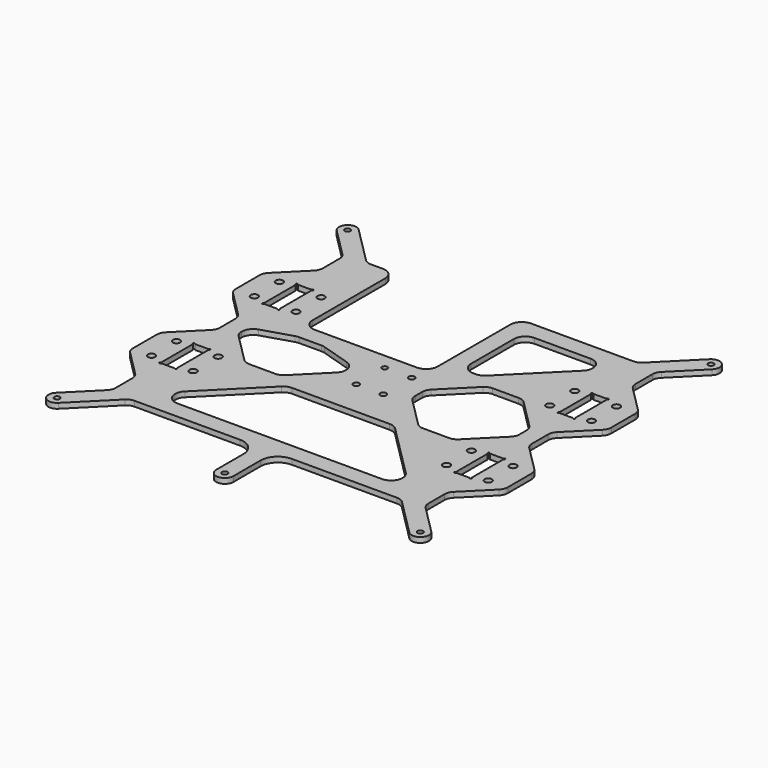
from build123d import *

# Parameters (mm, degrees)
F0_R     = 1.6
F0_R_2   = 2.1
F0_R_3   = 1.75
F1_DEPTH = 3


# Not quite as in the source:
# - ends of sketch curves that miss each other by under 0.0002 mm in the source are joined


with BuildPart() as f1:
    # F0 (on Top) → F1 (new body)
    with BuildSketch(Plane.XY):
        with BuildLine():
            Line((-91.7573578066, 64.2426430438), (-106.2426418066, 49.7573620438))
            ThreePointArc((-106.2426418066, 49.7573620438), (-107.5432800387, 47.8108195211), (-108.0000028014, 45.5147184321))
            Line((-108.0000028014, 45.5147184321), (-108.0000028014, 28.4852814321))
            ThreePointArc((-108.0000028014, 28.4852814321), (-107.5432780557, 26.1891807819), (-106.2426416956, 24.2426405379))
            Line((-106.2426416956, 24.2426405379), (-91.7573578066, 9.7573586489))
            ThreePointArc((-91.7573578066, 9.7573586489), (-90.4567263652, 7.8108163857), (-90.000004, 5.5147176489))
            Line((-90.000004, 5.5147176489), (-90.000004, -5.5147181357))
            ThreePointArc((-90.000004, -5.5147181357), (-90.4567266866, -7.810818842), (-91.7573628987, -9.7573592371))
            Line((-91.7573628987, -9.7573592371), (-106.2426418014, -24.2426401357))
            ThreePointArc((-106.2426418014, -24.2426401357), (-107.5432798474, -26.1891795848), (-108.0000028014, -28.4852801357))
            Line((-108.0000028014, -28.4852801357), (-108.0000028014, -45.5147181357))
            ThreePointArc((-108.0000028014, -45.5147181357), (-107.5432780557, -47.810818786), (-106.2426416956, -49.75735903))
            Line((-106.2426416956, -49.75735903), (-91.7573578014, -64.2426391357))
            ThreePointArc((-91.7573578014, -64.2426391357), (-90.4567259825, -66.1891833228), (-90.000004, -68.4852831357))
            Line((-90.000004, -68.4852831357), (-90.000004, -80.514722))
            ThreePointArc((-90.000004, -80.514722), (-90.4567219139, -82.8108200561), (-91.7573566058, -84.7573583942))
            Line((-91.7573566058, -84.7573583942), (-108.000003, -101.000004))
            ThreePointArc((-108.000003, -101.000004), (-107.9999999189, -107.9999994189), (-101.0000038311, -108.0000031689))
            Line((-101.0000038311, -108.0000031689), (-79.757363, -86.757362))
            ThreePointArc((-79.757363, -86.757362), (-77.8108216333, -85.4567247319), (-75.51472, -85.000001))
            Line((-75.51472, -85.000001), (-14.949748, -85.000001))
            ThreePointArc((-14.949748, -85.000001), (-7.8786801881, -87.9289331881), (-4.949748, -95.000001))
            Line((-4.949748, -95.000001), (-4.949747, -114.500004))
            ThreePointArc((-4.949747, -114.500004), (0, -119.449747), (4.949747, -114.500004))
            Line((4.949747, -114.500004), (4.949746, -95.000001))
            ThreePointArc((4.949746, -95.000001), (7.8786781881, -87.9289331881), (14.949746, -85.000001))
            Line((14.949746, -85.000001), (75.514718, -85.000001))
            ThreePointArc((75.514718, -85.000001), (77.8108209367, -85.4567226928), (79.7573623942, -86.7573616058))
            Line((79.7573623942, -86.7573616058), (101.000003, -108.000003))
            ThreePointArc((101.000003, -108.000003), (107.9999999189, -107.9999994189), (108.0000021689, -101.0000028311))
            Line((108.0000021689, -101.0000028311), (91.757279, -84.757281))
            ThreePointArc((91.757279, -84.757281), (90.4566428049, -82.8107405942), (89.99992, -80.51464))
            Line((89.99992, -80.51464), (89.99992, -68.9356846639))
            ThreePointArc((89.99992, -68.9356846639), (90.4566436949, -66.6395847167), (91.7572811413, -64.6930458052))
            Line((91.7572811413, -64.6930458052), (106.2425711968, -50.2077726639))
            ThreePointArc((106.2425711968, -50.2077726639), (107.5432095472, -48.2612339103), (107.9999341968, -45.9651336639))
            Line((107.9999341968, -45.9651336639), (107.9999501968, -28.9356956639))
            ThreePointArc((107.9999501968, -28.9356956639), (107.5432290112, -26.6395943825), (106.2425940052, -24.6930528554))
            Line((106.2425940052, -24.6930528554), (91.7573201968, -10.2077616639))
            ThreePointArc((91.7573201968, -10.2077616639), (90.4566900386, -8.261219774), (89.9999692559, -5.9651186639))
            Line((89.9999692559, -5.9651186639), (89.999978386, 5.514733204))
            ThreePointArc((89.999978386, 5.514733204), (90.4567025196, 7.8108314385), (91.7573390273, 9.7573687908))
            Line((91.7573390273, 9.7573687908), (106.2426308014, 24.2426424321))
            ThreePointArc((106.2426308014, 24.2426424321), (107.5432689605, 26.1891807238), (107.9999938014, 28.4852804321))
            Line((107.9999938014, 28.4852804321), (108.0000098014, 45.5147194321))
            ThreePointArc((108.0000098014, 45.5147194321), (107.5432888072, 47.8108202515), (106.2426536099, 49.7573622406))
            Line((106.2426536099, 49.7573622406), (91.7573798014, 64.2426534321))
            ThreePointArc((91.7573798014, 64.2426534321), (90.4567425354, 66.1891959193), (90.000022, 68.4852984321))
            Line((90.000022, 68.4852984321), (90.000022, 80.514742))
            ThreePointArc((90.000022, 80.514742), (90.4567448049, 82.8108425942), (91.7573813129, 84.7573826871))
            Line((91.7573813129, 84.7573826871), (108.000002, 101.000003))
            ThreePointArc((108.000002, 101.000003), (107.9999996689, 107.9999996689), (101.0000033311, 108.0000026689))
            Line((101.0000033311, 108.0000026689), (79.757362, 86.757362))
            ThreePointArc((79.757362, 86.757362), (77.8108201714, 85.4567245406), (75.514718, 85.000001))
            Line((75.514718, 85.000001), (16.5999989614, 85.000001))
            ThreePointArc((16.5999989614, 85.000001), (11.933094179, 83.0669057293), (9.9999989614, 78.400000925))
            Line((9.9999989614, 78.400000925), (9.9999993466, 26.100000075))
            ThreePointArc((9.9999993466, 26.100000075), (8.0669041289, 21.4330952707), (3.3999993466, 19.5))
            Line((3.3999993466, 19.5), (-55.3999990225, 19.5))
            ThreePointArc((-55.3999990225, 19.5), (-60.0669037518, 21.4330952177), (-61.9999990225, 26.099999925))
            Line((-61.9999990225, 26.099999925), (-61.9999996168, 78.3999997378))
            ThreePointArc((-61.9999996168, 78.3999997378), (-63.9330951112, 83.0669046688), (-68.6000002494, 84.9999996628))
            Line((-68.6000002494, 84.9999996628), (-75.5147185782, 84.999999))
            ThreePointArc((-75.5147185782, 84.999999), (-77.8108213035, 85.4567230195), (-79.7573624724, 86.7573621058))
            Line((-79.7573624724, 86.7573621058), (-101.000004, 108.000003))
            ThreePointArc((-101.000004, 108.000003), (-107.9999996689, 107.9999996689), (-108.0000031689, 101.0000038311))
            Line((-108.0000031689, 101.0000038311), (-91.757358, 84.757358))
            ThreePointArc((-91.757358, 84.757358), (-90.4567266686, 82.8108174694), (-90.000004, 80.514721))
            Line((-90.000004, 80.514721), (-90.000004, 68.4852860438))
            ThreePointArc((-90.000004, 68.4852860438), (-90.4567264392, 66.1891839348), (-91.7573578066, 64.2426430438))
        make_face()
        with Locations((-104.5, -104.5)):
            Circle(F0_R, mode=Mode.SUBTRACT)
        with Locations((-97, -45.9999990463)):
            Circle(F0_R_2, mode=Mode.SUBTRACT)
        with BuildLine():
            Line((-81.3660647171, -49.0500016357), (-88.6340257171, -49.0499986357))
            ThreePointArc((-88.6340257171, -49.0499986357), (-88.8840255651, -49.1169858461), (-89.0670382435, -49.2999983318))
            ThreePointArc((-89.0670382435, -49.2999983318), (-89.8536046247, -49.4035525093), (-89.750052771, -48.6169865423))
            ThreePointArc((-89.750052771, -48.6169865423), (-89.5670414944, -48.4339747338), (-89.5000547171, -48.1839756357))
            Line((-89.5000547171, -48.1839756357), (-89.5000547171, -25.8160226357))
            ThreePointArc((-89.5000547171, -25.8160226357), (-89.5670414944, -25.5660235377), (-89.7500529131, -25.3830109753))
            ThreePointArc((-89.7500529131, -25.3830109753), (-89.8536046247, -24.5964447622), (-89.0670389406, -24.6999987648))
            ThreePointArc((-89.0670389406, -24.6999987648), (-88.8840255651, -24.8830114254), (-88.6340257171, -24.9499986357))
            Line((-88.6340257171, -24.9499986357), (-81.3660647171, -24.9499956357))
            ThreePointArc((-81.3660647171, -24.9499956357), (-81.116065244, -24.8830086419), (-80.9330526237, -24.6999966897))
            ThreePointArc((-80.9330526237, -24.6999966897), (-80.1464875373, -24.5964460343), (-80.2500418461, -25.3830114122))
            ThreePointArc((-80.2500418461, -25.3830114122), (-80.4330543817, -25.5660245712), (-80.5000417171, -25.8160246357))
            Line((-80.5000417171, -25.8160246357), (-80.5000417171, -48.1839736357))
            ThreePointArc((-80.5000417171, -48.1839736357), (-80.4330543817, -48.4339737003), (-80.250041588, -48.6169864122))
            ThreePointArc((-80.250041588, -48.6169864122), (-80.1464878435, -49.4035515434), (-80.9330538105, -49.2999996897))
            ThreePointArc((-80.9330538105, -49.2999996897), (-81.116065619, -49.1169884131), (-81.3660647171, -49.0500016357))
        make_face(mode=Mode.SUBTRACT)
        with Locations((-73.000000298, -45.9999990016)):
            Circle(F0_R_2, mode=Mode.SUBTRACT)
        with Locations((-97, -27.9999990463)):
            Circle(F0_R_2, mode=Mode.SUBTRACT)
        with Locations((-73.000000298, -27.9999990016)):
            Circle(F0_R_2, mode=Mode.SUBTRACT)
        with BuildLine():
            ThreePointArc((28.066188, -31.000007), (30.591899845, -31.5024021647), (32.7330947558, -32.9331032442))
            Line((32.7330947558, -32.9331032442), (63.533094, -63.733105))
            ThreePointArc((63.533094, -63.733105), (64.9637917962, -70.9257175415), (58.866189, -75.000005))
            Line((58.866189, -75.000005), (-58.866192, -75.00001))
            ThreePointArc((-58.866192, -75.00001), (-64.9637994156, -70.9257194549), (-63.5330998772, -63.7331011228))
            Line((-63.5330998772, -63.7331011228), (-32.733097, -32.933104))
            ThreePointArc((-32.733097, -32.933104), (-30.5919024623, -31.5024030886), (-28.066191, -31.000008))
            Line((-28.066191, -31.000008), (28.066188, -31.000007))
        make_face(mode=Mode.SUBTRACT)
        with BuildLine():
            ThreePointArc((-24.6419521685, 3.9567877686), (-21.2857213242, 1.5678055586), (-20, -2.3460725892))
            Line((-20, -2.3460725892), (-20, -2.514719))
            ThreePointArc((-20, -2.514719), (-20.4567226696, -4.8108192675), (-21.7573588129, -6.7573591871))
            Line((-21.7573588129, -6.7573591871), (-38.242642, -23.242641))
            ThreePointArc((-38.242642, -23.242641), (-40.189182521, -24.543277657), (-42.485283, -25))
            Line((-42.485283, -25), (-57.51472, -25.000001))
            ThreePointArc((-57.51472, -25.000001), (-59.8108200561, -24.5432770037), (-61.7573596871, -23.2426406871))
            Line((-61.7573596871, -23.2426406871), (-78.242638, -6.75736))
            ThreePointArc((-78.242638, -6.75736), (-79.5432749414, -4.8108198087), (-79.999998, -2.514719))
            Line((-79.999998, -2.514719), (-79.999999, -2.3460724397))
            ThreePointArc((-79.999999, -2.3460724397), (-78.7142777333, 1.5678056301), (-75.3580470166, 3.9567878605))
            Line((-75.3580470166, 3.9567878605), (-58.4711977499, 9.2028603003))
            ThreePointArc((-58.4711977499, 9.2028603003), (-57.5033825389, 9.4252922533), (-56.5131497334, 9.5))
            Line((-56.5131497334, 9.5), (-43.4868514976, 9.5))
            ThreePointArc((-43.4868514976, 9.5), (-42.4966187879, 9.4252922678), (-41.5288036661, 9.2028603578))
            Line((-41.5288036661, 9.2028603578), (-24.6419521685, 3.9567877686))
        make_face(mode=Mode.SUBTRACT)
        with Locations((-7.7499998733, -10.25)):
            Circle(F0_R_3, mode=Mode.SUBTRACT)
        with Locations((0, -114.5)):
            Circle(F0_R, mode=Mode.SUBTRACT)
        with Locations((104.5, -104.5)):
            Circle(F0_R, mode=Mode.SUBTRACT)
        with Locations((7.7499998733, -10.25)):
            Circle(F0_R_3, mode=Mode.SUBTRACT)
        with Locations((72.9999979138, -46.2736748246)):
            Circle(F0_R_2, mode=Mode.SUBTRACT)
        with BuildLine():
            ThreePointArc((89.0668645807, -49.7150240159), (88.8838518688, -49.5320112222), (88.6338518043, -49.4650238868))
            Line((88.6338518043, -49.4650238868), (81.3658908043, -49.4650208868))
            ThreePointArc((81.3658908043, -49.4650208868), (81.1158917063, -49.5320076641), (80.9328791439, -49.7150190829))
            ThreePointArc((80.9328791439, -49.7150190829), (80.1463133184, -49.818569182), (80.2498686834, -49.0320036774))
            ThreePointArc((80.2498686834, -49.0320036774), (80.4328814689, -48.8489919513), (80.4998688043, -48.5989918868))
            Line((80.4998688043, -48.5989918868), (80.4998868043, -26.2310428868))
            ThreePointArc((80.4998868043, -26.2310428868), (80.4328996854, -25.9810431972), (80.2498874252, -25.7980305434))
            ThreePointArc((80.2498874252, -25.7980305434), (80.1463339307, -25.0114639792), (80.9328998977, -25.1150158329))
            ThreePointArc((80.9328998977, -25.1150158329), (81.1159118982, -25.2980276429), (81.3659108043, -25.3650148868))
            Line((81.3659108043, -25.3650148868), (88.6338718043, -25.3650238868))
            ThreePointArc((88.6338718043, -25.3650238868), (88.8838722193, -25.2980369264), (89.0668853307, -25.1150241907))
            ThreePointArc((89.0668853307, -25.1150241907), (89.8534511949, -25.0114714962), (89.7498988582, -25.7980369802))
            ThreePointArc((89.7498988582, -25.7980369802), (89.5668867982, -25.9810494138), (89.4998998043, -26.2310488868))
            Line((89.4998998043, -26.2310488868), (89.4998818043, -48.5990018868))
            ThreePointArc((89.4998818043, -48.5990018868), (89.5668685817, -48.8490009848), (89.7498800004, -49.0320135472))
            ThreePointArc((89.7498800004, -49.0320135472), (89.8534300995, -49.8185793727), (89.0668645807, -49.7150240159))
        make_face(mode=Mode.SUBTRACT)
        with Locations((96.9999979138, -46.2736748246)):
            Circle(F0_R_2, mode=Mode.SUBTRACT)
        with Locations((72.9999988043, -28.4058290639)):
            Circle(F0_R_2, mode=Mode.SUBTRACT)
        with Locations((96.9999988043, -28.4058290639)):
            Circle(F0_R_2, mode=Mode.SUBTRACT)
        with Locations((-97, 28.0000009537)):
            Circle(F0_R_2, mode=Mode.SUBTRACT)
        with BuildLine():
            Line((-89.5000770688, 25.8160239321), (-89.5000770688, 48.1839769321))
            ThreePointArc((-89.5000770688, 48.1839769321), (-89.5670640627, 48.4339764052), (-89.7500760149, 48.6169890255))
            ThreePointArc((-89.7500760149, 48.6169890255), (-89.853626847, 49.4035549351), (-89.0670615424, 49.3000012361))
            ThreePointArc((-89.0670615424, 49.3000012361), (-88.8840481333, 49.1169882675), (-88.6340480688, 49.0500009321))
            Line((-88.6340480688, 49.0500009321), (-81.3660870688, 49.0500039321))
            ThreePointArc((-81.3660870688, 49.0500039321), (-81.1160878123, 49.116990801), (-80.9330752254, 49.3000024452))
            ThreePointArc((-80.9330752254, 49.3000024452), (-80.1465098891, 49.4035535336), (-80.2500641979, 48.6169881557))
            ThreePointArc((-80.2500641979, 48.6169881557), (-80.4330767334, 48.4339749967), (-80.5000640688, 48.1839749321))
            Line((-80.5000640688, 48.1839749321), (-80.5000640688, 25.8160259321))
            ThreePointArc((-80.5000640688, 25.8160259321), (-80.4330767334, 25.5660258676), (-80.2500639397, 25.3830131557))
            ThreePointArc((-80.2500639397, 25.3830131557), (-80.1465101952, 24.5964480245), (-80.9330761622, 24.6999998782))
            ThreePointArc((-80.9330761622, 24.6999998782), (-81.1160881873, 24.8830112798), (-81.3660870688, 24.9499979321))
            Line((-81.3660870688, 24.9499979321), (-88.6340480688, 24.9500009321))
            ThreePointArc((-88.6340480688, 24.9500009321), (-88.8840481333, 24.8830135968), (-89.0670608452, 24.700000803))
            ThreePointArc((-89.0670608452, 24.700000803), (-89.853626847, 24.5964469292), (-89.7500758727, 25.3830125925))
            ThreePointArc((-89.7500758727, 25.3830125925), (-89.5670640627, 25.5660244591), (-89.5000770688, 25.8160239321))
        make_face(mode=Mode.SUBTRACT)
        with Locations((-97, 46.0000000894)):
            Circle(F0_R_2, mode=Mode.SUBTRACT)
        with Locations((-73.000000298, 28.0000008643)):
            Circle(F0_R_2, mode=Mode.SUBTRACT)
        with Locations((-73.000000298, 46)):
            Circle(F0_R_2, mode=Mode.SUBTRACT)
        with Locations((-7.75, 10.2500002831)):
            Circle(F0_R, mode=Mode.SUBTRACT)
        with Locations((-104.5, 104.5)):
            Circle(F0_R, mode=Mode.SUBTRACT)
        with Locations((7.75, 10.2500002831)):
            Circle(F0_R_3, mode=Mode.SUBTRACT)
        with BuildLine():
            ThreePointArc((42.485281, -25), (40.1891807325, -24.5432773304), (38.2426408129, -23.2426411871))
            Line((38.2426408129, -23.2426411871), (21.757358, -6.75736))
            ThreePointArc((21.757358, -6.75736), (20.4567217458, -4.8108196502), (19.999999, -2.514719))
            Line((19.999999, -2.514719), (19.999999, 2.514718))
            ThreePointArc((19.999999, 2.514718), (20.4567228049, 4.8108185942), (21.7573593129, 6.7573586871))
            Line((21.7573593129, 6.7573586871), (38.242641, 23.242641))
            ThreePointArc((38.242641, 23.242641), (40.1891810591, 24.5432774657), (42.485281, 25))
            Line((42.485281, 25), (57.51471, 24.999988))
            ThreePointArc((57.51471, 24.999988), (59.8108107084, 24.5432641591), (61.7573493942, 23.2426263942))
            Line((61.7573493942, 23.2426263942), (78.242613, 6.75733))
            ThreePointArc((78.242613, 6.75733), (79.5432487099, 4.8107885392), (79.99997, 2.514687))
            Line((79.99997, 2.514687), (79.999967, -2.51475))
            ThreePointArc((79.999967, -2.51475), (79.5432409023, -4.8108507316), (78.2426017729, -6.7573897729))
            Line((78.2426017729, -6.7573897729), (61.757311, -23.242657))
            ThreePointArc((61.757311, -23.242657), (59.8107691333, -24.5432910428), (57.514669, -25.000012))
            Line((57.514669, -25.000012), (42.485281, -25))
        make_face(mode=Mode.SUBTRACT)
        with Locations((72.9999979138, 28)):
            Circle(F0_R_2, mode=Mode.SUBTRACT)
        with Locations((73, 46)):
            Circle(F0_R_2, mode=Mode.SUBTRACT)
        with BuildLine():
            ThreePointArc((89.7499834183, 48.6169810255), (89.5669714661, 48.4339684052), (89.4999844722, 48.1839689321))
            Line((89.4999844722, 48.1839689321), (89.4999654722, 25.8160159321))
            ThreePointArc((89.4999654722, 25.8160159321), (89.5669524661, 25.5660164591), (89.7499644183, 25.3830038387))
            ThreePointArc((89.7499644183, 25.3830038387), (89.8535147675, 24.5964384462), (89.0669492628, 24.6999938112))
            ThreePointArc((89.0669492628, 24.6999938112), (88.8839359698, 24.8830063468), (88.6339364722, 24.9499939321))
            Line((88.6339364722, 24.9499939321), (81.3659754722, 24.9499969321))
            ThreePointArc((81.3659754722, 24.9499969321), (81.1159760237, 24.8830105298), (80.9329630618, 24.6999991691))
            ThreePointArc((80.9329630618, 24.6999991691), (80.1463981157, 24.5964485075), (80.2499526013, 25.3830137086))
            ThreePointArc((80.2499526013, 25.3830137086), (80.4329651369, 25.5660258676), (80.4999524722, 25.8160259321))
            Line((80.4999524722, 25.8160259321), (80.4999714722, 48.1839749321))
            ThreePointArc((80.4999714722, 48.1839749321), (80.4329841369, 48.4339749967), (80.2499713432, 48.6169877086))
            ThreePointArc((80.2499713432, 48.6169877086), (80.1464189049, 49.4035541459), (80.9329845656, 49.3000019861))
            ThreePointArc((80.9329845656, 49.3000019861), (81.1159959992, 49.116989926), (81.3659954722, 49.0500029321))
            Line((81.3659954722, 49.0500029321), (88.6339564722, 49.0499939321))
            ThreePointArc((88.6339564722, 49.0499939321), (88.8839565368, 49.1169812675), (89.0669692487, 49.2999940612))
            ThreePointArc((89.0669692487, 49.2999940612), (89.8535356861, 49.4035464995), (89.7499834183, 48.6169810255))
        make_face(mode=Mode.SUBTRACT)
        with Locations((96.9999988079, 28)):
            Circle(F0_R_2, mode=Mode.SUBTRACT)
        with Locations((97.0000008941, 46)):
            Circle(F0_R_2, mode=Mode.SUBTRACT)
        with BuildLine():
            ThreePointArc((32.7330950487, 32.9331039513), (30.5919004623, 31.5024030886), (28.066189, 31.000008))
            Line((28.066189, 31.000008), (26.599999425, 31.0000065721))
            ThreePointArc((26.599999425, 31.0000065721), (21.9330946957, 32.9331017897), (19.999999425, 37.6000064971))
            Line((19.999999425, 37.6000064971), (19.999999075, 68.4000096107))
            ThreePointArc((19.999999075, 68.4000096107), (21.9330942927, 73.066914843), (26.599999075, 75.0000101136))
            Line((26.599999075, 75.0000101136), (58.86619, 75.0000101136))
            ThreePointArc((58.86619, 75.0000101136), (64.9637974156, 70.9257194549), (63.5330978772, 63.7331011228))
            Line((63.5330978772, 63.7331011228), (32.7330950487, 32.9331039513))
        make_face(mode=Mode.SUBTRACT)
        with Locations((104.5, 104.5)):
            Circle(F0_R, mode=Mode.SUBTRACT)
    extrude(amount=F1_DEPTH)


solid = f1.part
